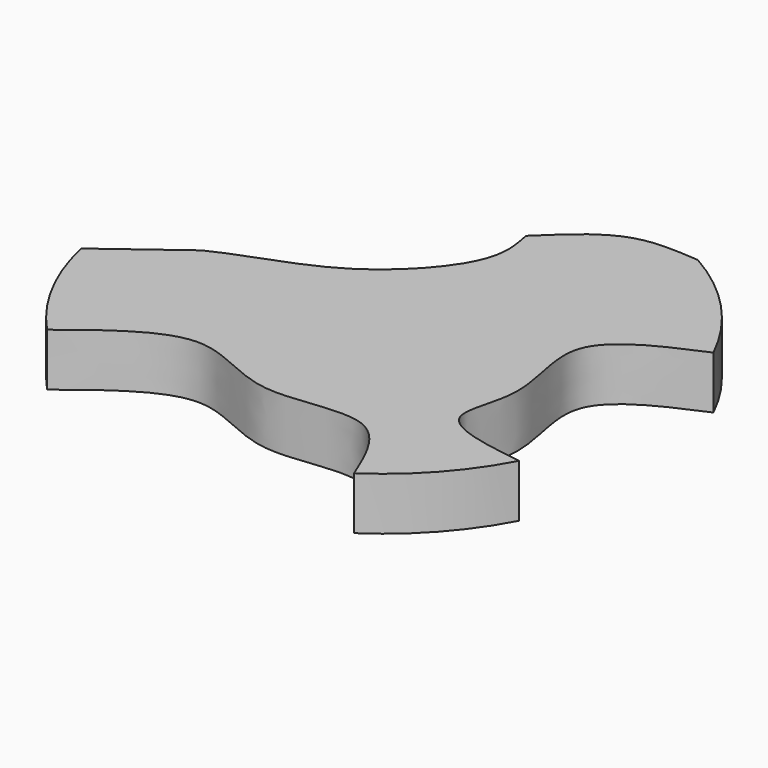
from build123d import *

# Parameters (mm, degrees)
F1_DEPTH = 5


with BuildPart() as f1:
    # F0 (on Top) → F1 (new body)
    with BuildSketch(Plane.XY):
        with BuildLine():
            add(Edge.make_bspline(
                [(22.5121691, 10.8720854676), (18.8895611428, 9.3055197167), (11.9102659407, 6.2896821538), (16.4364178682, -3.0658471403), (12.2521680449, -10.2063529762), (18.6615851191, -11.1474987265), (22.1188925873, -11.6513772023)],
                knots=[0, 0, 0, 0, 0.2780136343, 0.5343531988, 0.7479805585, 1, 1, 1, 1], degree=3))
            ThreePointArc((22.5121691, 10.8720854676), (18.2564856156, 17.0792486067), (12.34633467, 21.7386296766))
            add(Edge.make_bspline(
                [(0, 16.8172493577), (1.9144161531, 18.6824676113), (5.5934798745, 22.2645311542), (10.1584208321, 21.9120162799), (12.34633467, 21.7386296766)],
                knots=[0, 0, 0, 0, 0.5203475383, 1, 1, 1, 1], degree=3))
            add(Edge.make_bspline(
                [(0, 12.2895278037), (0.5700685894, 13.9777110398), (0.2850342947, 15.3974801988), (0, 16.8172493577)],
                knots=[0.8181160828, 0.8181160828, 0.8181160828, 0.8181160828, 1, 1, 1, 1], degree=3))
            add(Edge.make_bspline(
                [(-17.3023622483, 0), (-14.1903788127, 1.5720662607), (-6.6472654424, 3.2397841474), (-0.8648455283, 9.7284013886), (0, 12.2895278037)],
                knots=[0.254891956, 0.254891956, 0.254891956, 0.254891956, 0.542181756, 0.8181160828, 0.8181160828, 0.8181160828, 0.8181160828], degree=3))
            Line((-17.3023622483, 0), (-24.4273769181, -5.3200805351))
            ThreePointArc((-24.4273769181, -5.3200805351), (-22.1428727527, -11.6057393672), (-18.2737018092, -17.0608271249))
            add(Edge.make_bspline(
                [(-18.2737018092, -17.0608271249), (-14.8332101277, -14.3400323801), (-8.3808524987, -9.228978734), (-0.4412585546, -15.998889193), (10.2263751779, -12.0238586347), (12.6576888155, -17.9664290501), (13.8278126154, -20.8276642539)],
                knots=[0, 0, 0, 0, 0.2769679297, 0.5181649262, 0.767240907, 1, 1, 1, 1], degree=3))
            ThreePointArc((13.8278126154, -20.8276642539), (18.549729506, -16.7602963951), (22.1188925873, -11.6513772023))
        make_face()
    extrude(amount=F1_DEPTH)


solid = f1.part
